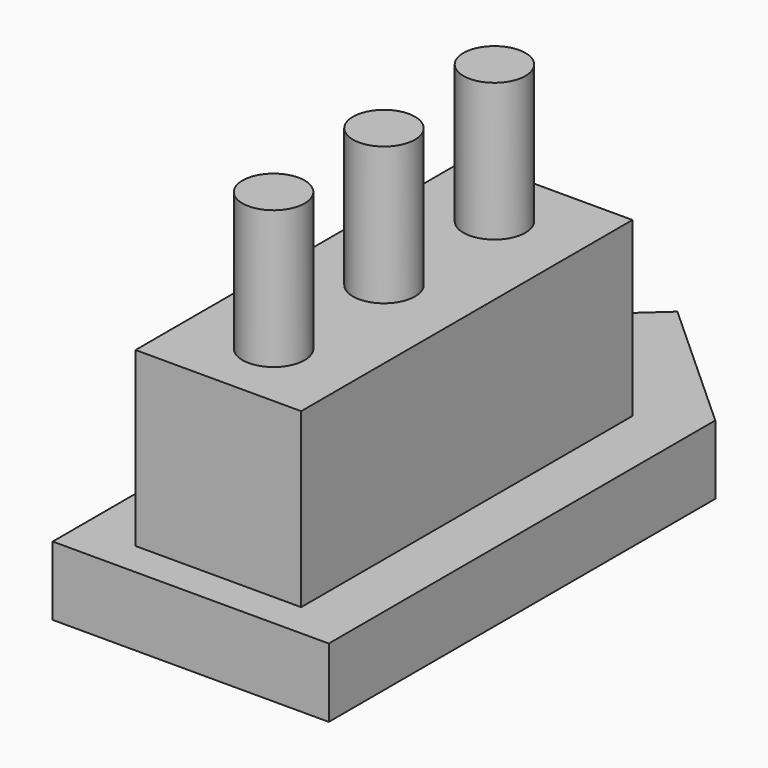
from build123d import *

# Parameters (mm, degrees)
F1_DEPTH     = 10
F2_W         = 24
F2_H         = 60
F3_DEPTH     = 25
F4_R         = 4.5
F5_DEPTH     = 20
F6_TEXT_SIZE = 11.1111111111
F7_DEPTH     = 2.5


# Not quite as in the source:
# - Text() gives the source's letters only with a copy of the font that has no kerning and outlines rounded to 1/6400 em; it was checked with that copy


with BuildPart() as f1:
    # F0 (on Top) → F1 (new body)
    with BuildSketch(Plane.XY):
        Polygon((-20, -35), (20, -35), (20, 35), (0, 53.1383571472), (-20, 35), align=None)
    extrude(amount=F1_DEPTH)

    # F2 (on face) → F3 (join)
    with BuildSketch(Plane.XY.offset(10)):
        Rectangle(F2_W, F2_H)
    extrude(amount=F3_DEPTH)

    # F4 (on face) → F5 (join)
    with BuildSketch(Plane.XY.offset(35)):
        with Locations((0, -20)):
            Circle(F4_R)
        Circle(F4_R)
        with Locations((0, 20)):
            Circle(F4_R)
    extrude(amount=F5_DEPTH)

    # F6 (on face) → F7 (join)
    with BuildSketch(Plane(origin=(-12, 0, 0), x_dir=(0, -1, 0), z_dir=(-1, 0, 0))):
        with Locations((-25.9151100771, 18.5699017233)):
            Text('f.abdullah', F6_TEXT_SIZE, font='Open Sans', text_align=(TextAlign.LEFT, TextAlign.BOTTOM))
    extrude(amount=F7_DEPTH)


solid = f1.part
